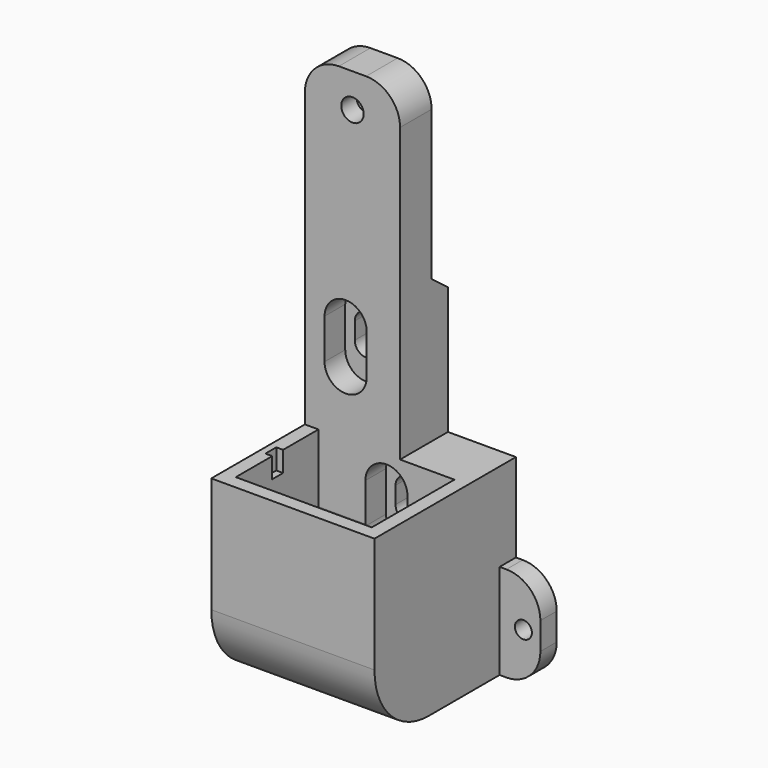
from build123d import *

# Parameters (mm, degrees)
F0_W         = 24
F0_H         = 26
F1_DEPTH     = 27
F2_W         = 20
F2_H         = 15.2
F3_DEPTH     = 25
F4_W         = 20
F4_H         = 10
F5_DEPTH     = 24
F7_W         = 3
F7_H         = 14
F8_DEPTH     = 6
F6_W         = 3
F6_H         = 14
F9_DEPTH     = 6
F10_R        = 1.25
F11_DEPTH    = 3
F12_R        = 5
F14_DEPTH    = 48
F15_W        = 3
F15_H        = 30
F16_DEPTH    = 14
F17_T4_DEPTH = 14
F18_R        = 1.65
F19_DEPTH    = 5.8
F21_DEPTH    = 3
F23_DEPTH    = 8.8
F24_DEPTH    = 5
F25_R        = 10
F26_T1_DEPTH = 20
F27_W        = 1
F27_H        = 2
F28_DEPTH    = 3
F29_R        = 5


# Not quite as in the source:
# - a fillet or chamfer that OpenCascade refuses, or shapes differently, is made with other operations: its cross-section is extruded or revolved along the edge and cut away or added


with BuildPart() as f1:
    # F0 (on Top) → F1 (new body)
    with BuildSketch(Plane.XY):
        Rectangle(F0_W, F0_H)
    extrude(amount=F1_DEPTH)

    # F2 (on face) → F3 (cut)
    with BuildSketch(Plane.XY.offset(27)):
        with Locations((0, -3.4)):
            Rectangle(F2_W, F2_H)
    extrude(amount=-F3_DEPTH, mode=Mode.SUBTRACT)

    # F4 (on face) → F5 (cut, through all)
    with BuildSketch(Plane(origin=(0, 13, 0), x_dir=(-1, 0, 0), z_dir=(0, 1, 0))):
        with Locations((0, 7)):
            Rectangle(F4_W, F4_H)
    extrude(amount=-F5_DEPTH, mode=Mode.SUBTRACT)

    # F7 (on face) → F8 (join)
    with BuildSketch(Plane.YZ.offset(12)):
        with Locations((11.5, 7)):
            Rectangle(F7_W, F7_H)
    extrude(amount=F8_DEPTH)

    # F6 (on face) → F9 (join)
    with BuildSketch(Plane(origin=(-12, 0, 0), x_dir=(0, -1, 0), z_dir=(-1, 0, 0))):
        with Locations((-11.5, 7)):
            Rectangle(F6_W, F6_H)
    extrude(amount=F9_DEPTH)

    # F10 (on face) → F11 (cut, through all)
    with BuildSketch(Plane(origin=(0, 13, 0), x_dir=(-1, 0, 0), z_dir=(0, 1, 0))):
        with Locations((-15.5, 7)):
            Circle(F10_R)
        with Locations((15.5, 7)):
            Circle(F10_R)
    extrude(amount=-F11_DEPTH, mode=Mode.SUBTRACT)

    # F12
    f12_edges = [f1.edges().sort_by_distance(p)[0] for p in [
        (18, 11.5, 14),
        (18, 11.5, 0),
        (-18, 11.5, 14),
        (-18, 11.5, 0),
    ]]
    fillet(f12_edges, radius=F12_R)

    # F13 (on face) → F14 (join)
    with BuildSketch(Plane.XY.offset(27)):
        Polygon((2, 13), (-12, 13), (-12, 4.2), (-10, 4.2), (2, 4.2), align=None)
    extrude(amount=F14_DEPTH)

    # F15 (on face) → F16 (cut, through all)
    with BuildSketch(Plane(origin=(-12, 0, 0), x_dir=(0, -1, 0), z_dir=(-1, 0, 0))):
        with Locations((-11.5, 60)):
            Rectangle(F15_W, F15_H)
    extrude(amount=-F16_DEPTH, mode=Mode.SUBTRACT)

    # F17: chamfer of 3 x 4 on 1 edges, made by hand


with BuildPart() as f17_tool2:
    # F17_s3 → F17_t4 (new body)
    with BuildSketch(Plane.YZ.offset(-12)):
        Polygon((14, 45), (10, 48), (10, 45), align=None)
    extrude(amount=F17_T4_DEPTH)

    split(bisect_by=Plane.XZ.offset(-13), keep=Keep.TOP)


with BuildPart() as f1_1:
    add(f1.part)

    # F17_t1: union F17_tool2
    add(f17_tool2.part)

    # F18 (on face) → F19 (cut, through all)
    with BuildSketch(Plane.XZ.offset(-4.2)):
        with Locations((-5, 70)):
            Circle(F18_R)
    extrude(amount=-F19_DEPTH, mode=Mode.SUBTRACT)

    # F20 (on face) → F21 (cut)
    with BuildSketch(Plane(origin=(0, 10, 0), x_dir=(-1, 0, 0), z_dir=(0, 1, 0))):
        Polygon((8.4994896827, 70.0597658786), (6.6979860722, 73.0605299049), (3.1984963894, 73.0007640263), (1.5005103171, 69.9402341215), (3.3020139276, 66.9394700952), (6.8015036104, 66.9992359738), align=None)
    extrude(amount=-F21_DEPTH, mode=Mode.SUBTRACT)

    # F22 (on face) → F23 (cut, through all)
    with BuildSketch(Plane(origin=(0, 13, 0), x_dir=(-1, 0, 0), z_dir=(0, 1, 0))):
        with BuildLine():
            ThreePointArc((3.1, 22.625), (0, 25.725), (-3.1, 22.625))
            Line((-3.1, 22.625), (-3.1, 16.725))
            ThreePointArc((-3.1, 16.725), (0, 13.625), (3.1, 16.725))
            Line((3.1, 16.725), (3.1, 22.625))
        make_face()
        with BuildLine():
            Line((1.7, 20.925), (1.7, 18.425))
            ThreePointArc((1.7, 18.425), (1.202081528, 17.222918472), (0, 16.725))
            ThreePointArc((0, 16.725), (-1.202081528, 17.222918472), (-1.7, 18.425))
            Line((-1.7, 18.425), (-1.7, 20.925))
            ThreePointArc((-1.7, 20.925), (-1.202081528, 22.127081528), (0, 22.625))
            ThreePointArc((0, 22.625), (1.202081528, 22.127081528), (1.7, 20.925))
        make_face(mode=Mode.SUBTRACT)
        with BuildLine():
            ThreePointArc((9.1, 41.95), (6, 45.05), (2.9, 41.95))
            Line((2.9, 41.95), (2.9, 36.05))
            ThreePointArc((2.9, 36.05), (6, 32.95), (9.1, 36.05))
            Line((9.1, 36.05), (9.1, 41.95))
        make_face()
        with BuildLine():
            ThreePointArc((4.3, 40.25), (4.797918472, 41.452081528), (6, 41.95))
            ThreePointArc((6, 41.95), (7.202081528, 41.452081528), (7.7, 40.25))
            Line((7.7, 40.25), (7.7, 37.75))
            ThreePointArc((7.7, 37.75), (7.202081528, 36.547918472), (6, 36.05))
            ThreePointArc((6, 36.05), (4.797918472, 36.547918472), (4.3, 37.75))
            Line((4.3, 37.75), (4.3, 40.25))
        make_face(mode=Mode.SUBTRACT)
        with BuildLine():
            ThreePointArc((-1.7, 18.425), (-1.202081528, 17.222918472), (0, 16.725))
            Line((0, 16.725), (0, 22.625))
            ThreePointArc((0, 22.625), (-1.202081528, 22.127081528), (-1.7, 20.925))
            Line((-1.7, 20.925), (-1.7, 18.425))
        make_face()
        with BuildLine():
            ThreePointArc((0, 16.725), (1.202081528, 17.222918472), (1.7, 18.425))
            Line((1.7, 18.425), (1.7, 20.925))
            ThreePointArc((1.7, 20.925), (1.202081528, 22.127081528), (0, 22.625))
            Line((0, 22.625), (0, 16.725))
        make_face()
        with BuildLine():
            Line((6, 41.95), (6, 40.25))
            Line((6, 40.25), (6, 37.75))
            Line((6, 37.75), (6, 36.05))
            ThreePointArc((6, 36.05), (7.202081528, 36.547918472), (7.7, 37.75))
            Line((7.7, 37.75), (7.7, 40.25))
            ThreePointArc((7.7, 40.25), (7.202081528, 41.452081528), (6, 41.95))
        make_face()
        with BuildLine():
            Line((6, 37.75), (6, 40.25))
            Line((6, 40.25), (6, 41.95))
            ThreePointArc((6, 41.95), (4.797918472, 41.452081528), (4.3, 40.25))
            Line((4.3, 40.25), (4.3, 37.75))
            ThreePointArc((4.3, 37.75), (4.797918472, 36.547918472), (6, 36.05))
            Line((6, 36.05), (6, 37.75))
        make_face()
    extrude(amount=-F23_DEPTH, mode=Mode.SUBTRACT)

    # F22 (on face) → F24 (join)
    with BuildSketch(Plane(origin=(0, 13, 0), x_dir=(-1, 0, 0), z_dir=(0, 1, 0))):
        with BuildLine():
            ThreePointArc((3.1, 22.625), (0, 25.725), (-3.1, 22.625))
            Line((-3.1, 22.625), (-3.1, 16.725))
            ThreePointArc((-3.1, 16.725), (0, 13.625), (3.1, 16.725))
            Line((3.1, 16.725), (3.1, 22.625))
        make_face()
        with BuildLine():
            Line((1.7, 20.925), (1.7, 18.425))
            ThreePointArc((1.7, 18.425), (1.202081528, 17.222918472), (0, 16.725))
            ThreePointArc((0, 16.725), (-1.202081528, 17.222918472), (-1.7, 18.425))
            Line((-1.7, 18.425), (-1.7, 20.925))
            ThreePointArc((-1.7, 20.925), (-1.202081528, 22.127081528), (0, 22.625))
            ThreePointArc((0, 22.625), (1.202081528, 22.127081528), (1.7, 20.925))
        make_face(mode=Mode.SUBTRACT)
        with BuildLine():
            ThreePointArc((9.1, 41.95), (6, 45.05), (2.9, 41.95))
            Line((2.9, 41.95), (2.9, 36.05))
            ThreePointArc((2.9, 36.05), (6, 32.95), (9.1, 36.05))
            Line((9.1, 36.05), (9.1, 41.95))
        make_face()
        with BuildLine():
            ThreePointArc((4.3, 40.25), (4.797918472, 41.452081528), (6, 41.95))
            ThreePointArc((6, 41.95), (7.202081528, 41.452081528), (7.7, 40.25))
            Line((7.7, 40.25), (7.7, 37.75))
            ThreePointArc((7.7, 37.75), (7.202081528, 36.547918472), (6, 36.05))
            ThreePointArc((6, 36.05), (4.797918472, 36.547918472), (4.3, 37.75))
            Line((4.3, 37.75), (4.3, 40.25))
        make_face(mode=Mode.SUBTRACT)
    extrude(amount=-F24_DEPTH)

    # F25
    f25_edges = [f1_1.edges().sort_by_distance(p)[0] for p in [
        (0, -13, 0),
        (0, -11, 2),
    ]]
    fillet(f25_edges, radius=F25_R)

    # F26: fillet of radius 5 on 1 edges, made by hand

    # F26_s2 → F26_t1 (cut)
    with BuildSketch(Plane.YZ.offset(-10)):
        with BuildLine():
            ThreePointArc((4.2, 17), (5.6644660941, 13.4644660941), (9.2, 12))
            Line((9.2, 12), (4.2, 12))
            Line((4.2, 12), (4.2, 17))
        make_face()
    extrude(amount=F26_T1_DEPTH, mode=Mode.SUBTRACT)

    # F27 (on face) → F28 (cut)
    with BuildSketch(Plane.XY.offset(27)):
        with Locations((-10.5, -3.3)):
            Rectangle(F27_W, F27_H)
    extrude(amount=-F28_DEPTH, mode=Mode.SUBTRACT)

    # F29
    f29_edges = [f1_1.edges().sort_by_distance(p)[0] for p in [
        (-12, 7.1, 75),
        (2, 7.1, 75),
    ]]
    fillet(f29_edges, radius=F29_R)


solid = f1_1.part
